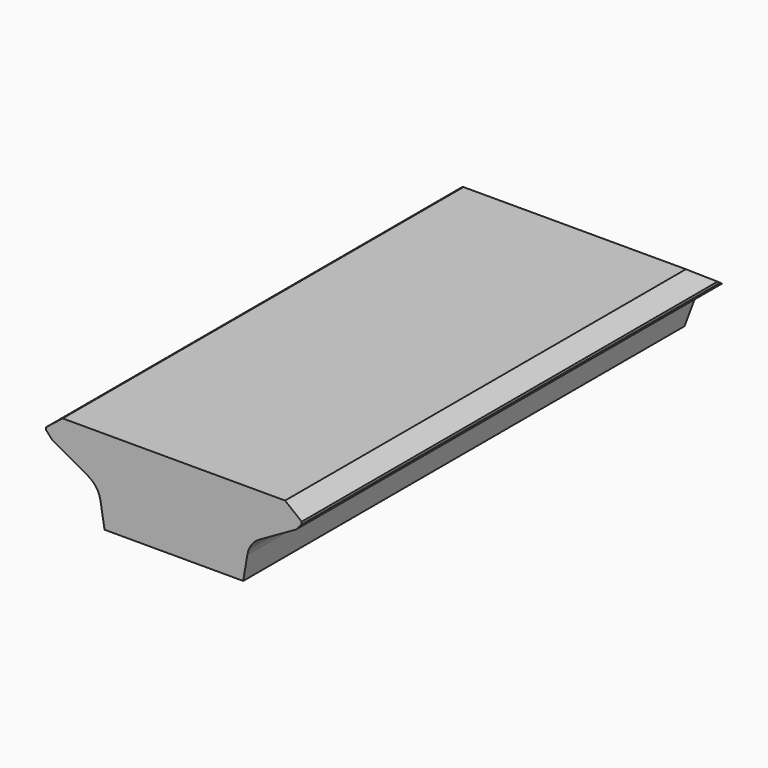
from build123d import *

# Parameters (mm, degrees)
F1_DEPTH    = 459.4
F2_SIZE2    = 31.5
F2_SIZE     = 11.8
F3_T1_DEPTH = 453.6970794399
F4_R        = 20


# Not quite as in the source:
# - a fillet or chamfer that OpenCascade refuses, or shapes differently, is made with other operations: its cross-section is extruded or revolved along the edge and cut away or added


with BuildPart() as f1:
    # F0 (on Front) → F1 (new body)
    with BuildSketch(Plane.XZ):
        Polygon((-61.18, 29.2), (-56.25, 0), (56.25, 0), (61.18, 29.2), (99, 50.6), (103.7, 55.8), (103.7, 57.8), (90.23, 68.48), (-90.23, 68.48), (-103.7, 57.8), (-103.7, 55.8), (-99, 50.6), align=None)
    extrude(amount=F1_DEPTH)

    # F2
    f2_edges = [f1.edges().sort_by_distance(p)[0] for p in [
        (0, 0, 0),
    ]]
    f2_side = f1.faces().sort_by_distance((0, -229.7, 0))[0]
    chamfer(f2_edges, length=F2_SIZE, length2=F2_SIZE2, reference=f2_side)

    # F3: chamfer of 52.9 x 37 on 1 edges, made by hand

    # F3_s2 → F3_t1 (cut)
    with BuildSketch(Plane.YZ.offset(-226.8485397199)):
        Polygon((0, 31.48), (-52.9, 68.48), (0, 68.48), align=None)
    extrude(amount=F3_T1_DEPTH, mode=Mode.SUBTRACT)

    # F4 (call 1 of 2: OpenCascade refuses the feature's edges together)
    f4_edges = [f1.edges().sort_by_distance(p)[0] for p in [
        (61.18, -230.130794, 29.2),
    ]]
    fillet(f4_edges, radius=F4_R)

    # F4#2 (call 2 of 2)
    f4_2_edges = [f1.edges().sort_by_distance(p)[0] for p in [
        (-61.18, -230.130794, 29.2),
    ]]
    fillet(f4_2_edges, radius=F4_R)


solid = f1.part
